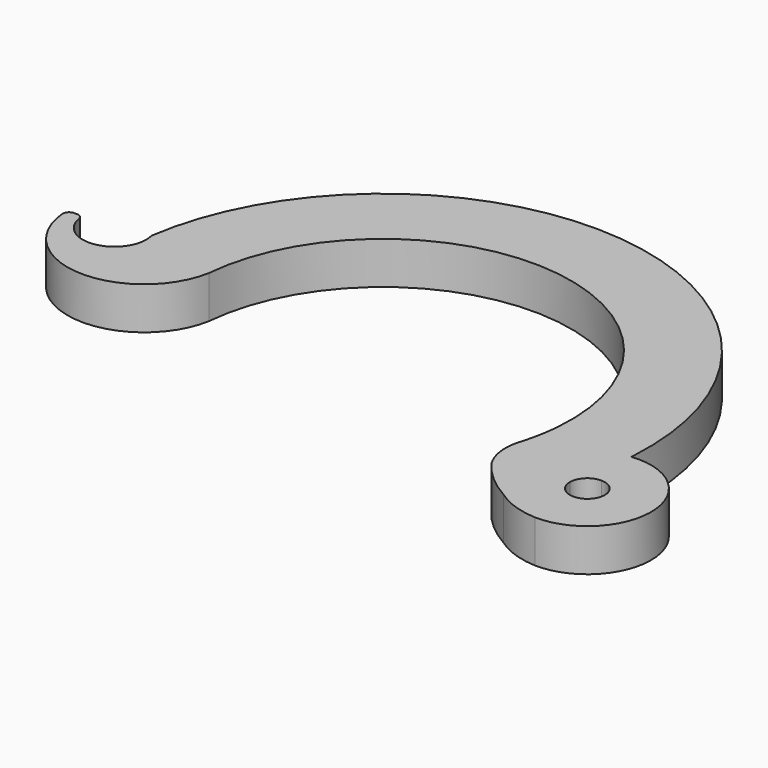
from build123d import *

# Parameters (mm, degrees)
F1_DEPTH = 20
F2_R     = 3


# Not quite as in the source:
# - a feature names something its author has since deleted; it is built from what else it names


with BuildPart() as f1:
    # F0 (on Top) → F1 (new body)
    with BuildSketch(Plane.XY):
        with BuildLine():
            Line((-153.2121218782, 14.4520842503), (-160.3632725747, 14.4520842503))
            ThreePointArc((-160.3632725747, 14.4520842503), (-127.3979918157, -21.6045066339), (-88.538816916, 8.0054918097))
            ThreePointArc((-88.538816916, 8.0054918097), (7.672936475, 88.5682564232), (88.5964468438, -7.3402729282))
            ThreePointArc((88.5964468438, -7.3402729282), (87.9631543537, -12.872197798), (86.984793992, -18.3536267309))
            ThreePointArc((86.984793992, -18.3536267309), (86.0838715562, -22.1985823397), (85.013080464, -25.9997336529))
            ThreePointArc((85.013080464, -25.9997336529), (84.2979595084, -36.2275225271), (87.887852798, -45.8312577069))
            ThreePointArc((87.887852798, -45.8312577069), (96.3394016955, -54.8865279313), (106.4780767567, -62.0022756507))
            ThreePointArc((106.4780767567, -62.0022756507), (116.2685705091, -67.06105094), (127.0920702884, -69.1339300658))
            ThreePointArc((127.0920702884, -69.1339300658), (157.854119606, -37.8760326334), (124.6599386157, -9.2141035549))
            ThreePointArc((124.6599386157, -9.2141035549), (124.7149682754, -8.4366277665), (124.7651490421, -7.6588239637))
            ThreePointArc((124.7651490421, -7.6588239637), (12.9161691706, 124.330899514), (-123.675215649, 18.1505105758))
            ThreePointArc((-123.675215649, 18.1505105758), (-136.3484686697, -0.431692042), (-153.2121218782, 14.4520842503))
        make_face()
        with BuildLine():
            ThreePointArc((127.83052, -30.8446834837), (133.6641509448, -33.2610525389), (136.08052, -39.0946834837))
            ThreePointArc((136.08052, -39.0946834837), (133.6641509448, -44.9283144285), (127.83052, -47.3446834837))
            ThreePointArc((127.83052, -47.3446834837), (121.9968890552, -44.9283144285), (119.58052, -39.0946834837))
            ThreePointArc((119.58052, -39.0946834837), (121.9968890552, -33.2610525389), (127.83052, -30.8446834837))
        make_face(mode=Mode.SUBTRACT)
    extrude(amount=F1_DEPTH)

    # F2
    f2_edges = [f1.edges().sort_by_distance(p)[0] for p in [
        (-160.363273, 14.452084, 10),
        (-153.212122, 14.452084, 10),
    ]]
    fillet(f2_edges, radius=F2_R)


solid = f1.part
